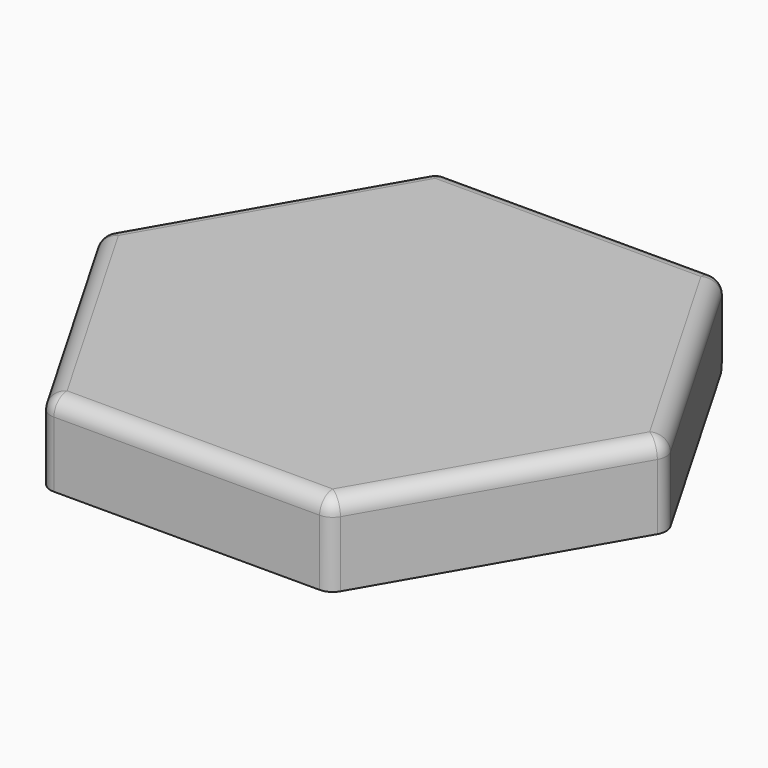
from build123d import *

# Parameters (mm, degrees)
F1_DEPTH  = 25.4
F2_R      = 5.08
F3_T      = -6.35
F4_R      = 3.175
F5_DEPTH  = 38.1
F8_DEPTH  = 87.2033022895
F9_R      = 3.175
F10_DEPTH = 87.2033022895
F11_R     = 2.54
F12_DEPTH = 38.1


# Not quite as in the source:
# - the program builds the solid bodies; features that only make, move or delete a surface that nothing else refers to are left out


with BuildPart() as f1:
    # F0 (on Top) → F1 (new body)
    with BuildSketch(Plane.XY):
        Polygon((-43.9940905122, -76.2), (43.9940905122, -76.2), (87.9881810245, 0), (43.9940905122, 76.2), (-43.9940905122, 76.2), (-87.9881810245, 0), align=None)
    extrude(amount=F1_DEPTH)

    # F2
    f2_edges = [f1.edges().sort_by_distance(p)[0] for p in [
        (-65.991136, -38.1, 25.4),
        (0, -76.2, 25.4),
        (65.991136, -38.1, 25.4),
        (65.991136, 38.1, 25.4),
        (0, 76.2, 25.4),
        (-65.991136, 38.1, 25.4),
        (43.994091, -76.2, 12.7),
        (87.988181, 0, 12.7),
        (-43.994091, -76.2, 12.7),
        (43.994091, 76.2, 12.7),
        (-43.994091, 76.2, 12.7),
        (-87.988181, 0, 12.7),
    ]]
    fillet(f2_edges, radius=F2_R)

    # F3
    f3_openings = [f1.faces().sort_by_distance(p)[0] for p in [
        (0, 0, 0),
    ]]
    offset(amount=F3_T, openings=f3_openings)

    # F4 (on Right) → F5 (join)
    with BuildSketch(Plane.YZ):
        with Locations((76.2, 0)):
            Circle(F4_R)
    extrude(amount=-F5_DEPTH)

    # F8 (cut, through all): a face of the model
    f8_faces = [f1.faces().sort_by_distance(p)[0] for p in [
        (0, 76.6491706172, -0.4491706172),
    ]]
    extrude(f8_faces, amount=F8_DEPTH, mode=Mode.SUBTRACT)

    # F9 (on face) → F10 (cut, through all)
    with BuildSketch(Plane.YZ):
        with Locations((76.2, 0)):
            Circle(F9_R)
    extrude(amount=F10_DEPTH, mode=Mode.SUBTRACT)

    # F11 (on face) → F12 (join)
    with BuildSketch(Plane.YZ):
        with Locations((76.2, 0)):
            Circle(F11_R)
    extrude(amount=F12_DEPTH)


solid = f1.part
